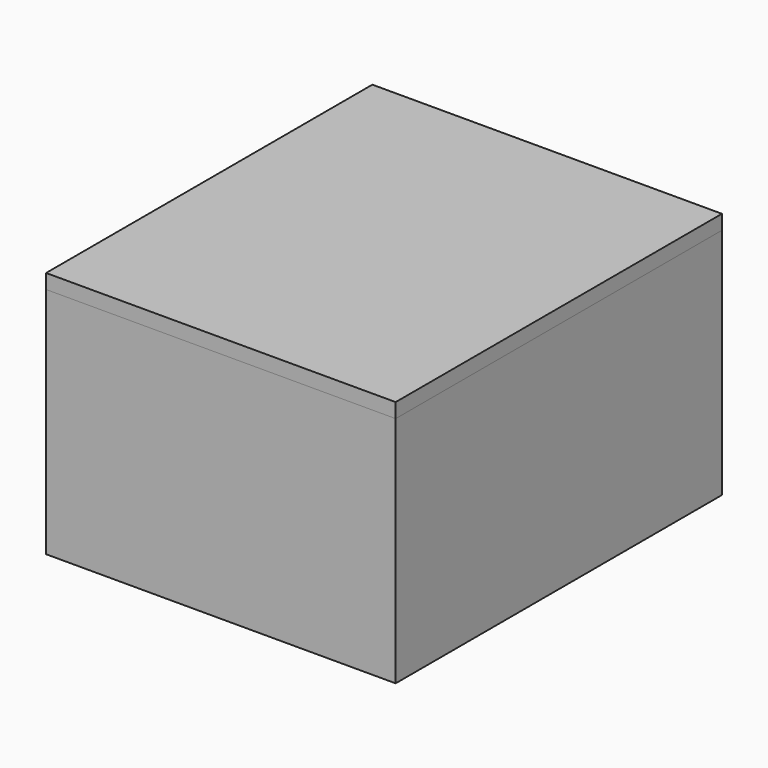
from build123d import *

# Parameters (mm, degrees)
F0_W     = 60
F0_H     = 70
F1_DEPTH = 40
F2_T     = -2.5
F3_W     = 60
F3_H     = 70
F3_W_2   = 55
F3_H_2   = 65
F4_DEPTH = 2.5
F5_DEPTH = 4
F6_R     = 2.5
F6_R_2   = 1.65
F7_DEPTH = 20


with BuildPart() as f1:
    # F0 (on Top) → F1 (new body)
    with BuildSketch(Plane.XY):
        Rectangle(F0_W, F0_H)
    extrude(amount=F1_DEPTH)

    # F2
    f2_openings = [f1.faces().sort_by_distance(p)[0] for p in [
        (0, 0, 40),
    ]]
    offset(amount=F2_T, openings=f2_openings)

    # F6 (on face) → F7 (join)
    with BuildSketch(Plane.XY.offset(2.5)):
        with Locations((-21.5, 26.5)):
            Circle(F6_R)
        with Locations((-21.5, 26.5)):
            Circle(F6_R_2, mode=Mode.SUBTRACT)
        with Locations((21.5, 26.5)):
            Circle(F6_R)
        with Locations((21.5, 26.5)):
            Circle(F6_R_2, mode=Mode.SUBTRACT)
        with Locations((-21.5, -29.5)):
            Circle(F6_R)
        with Locations((-21.5, -29.5)):
            Circle(F6_R_2, mode=Mode.SUBTRACT)
        with Locations((10, -29.5)):
            Circle(F6_R)
        with Locations((10, -29.5)):
            Circle(F6_R_2, mode=Mode.SUBTRACT)
    extrude(amount=F7_DEPTH)


with BuildPart() as f4:
    # F3 (on face) → F4 (new body)
    with BuildSketch(Plane.XY.offset(40)):
        Rectangle(F3_W, F3_H)
        Rectangle(F3_W_2, F3_H_2, mode=Mode.SUBTRACT)
        Rectangle(F3_W_2, F3_H_2)
    extrude(amount=F4_DEPTH)

    # F3 (on face) → F5 (join)
    with BuildSketch(Plane.XY.offset(40)):
        Rectangle(F3_W_2, F3_H_2)
    extrude(amount=-F5_DEPTH)


solid = Compound([f1.part, f4.part])
